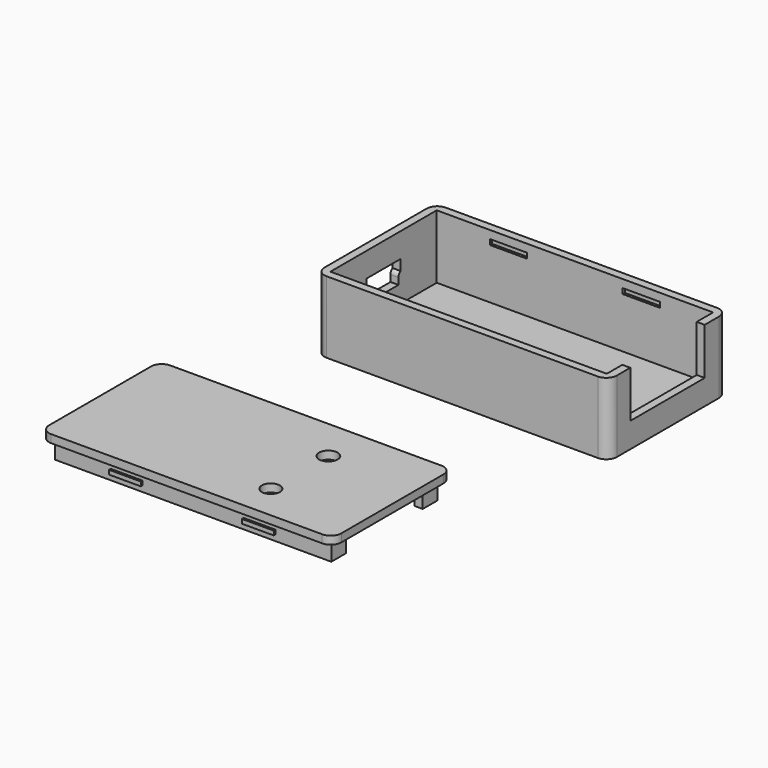
from build123d import *

# Parameters (mm, degrees)
F0_W        = 52
F0_H        = 25
F0_R        = 1.75
F1_DEPTH    = 1.5
F2_DEPTH    = 13.5
F3_W        = 17.5
F3_H        = 8.8
F4_DEPTH    = 25
F5_W        = 7
F5_H        = 2.1
F6_DEPTH    = 2
F7_T1_DEPTH = 5.8301270189
F9_W        = 7
F9_H        = 1
F10_DEPTH   = 0.5
F11_W       = 7
F11_H       = 1
F12_DEPTH   = 0.5
F0_R_2      = 1.7
F0_W_2      = 1.5
F0_H_2      = 18
F13_DEPTH   = 1.5
F14_DEPTH   = 5
F15_W       = 6
F15_H       = 0.8
F16_DEPTH   = 0.4
F17_W       = 6
F17_H       = 0.8
F18_DEPTH   = 0.5


# Not quite as in the source:
# - a fillet or chamfer that OpenCascade refuses, or shapes differently, is made with other operations: its cross-section is extruded or revolved along the edge and cut away or added


with BuildPart() as f1:
    # F0 (on Top) → F1 (new body)
    with BuildSketch(Plane.XY):
        Rectangle(F0_W, F0_H)
        with Locations((-21.9428632408, 0)):
            Circle(F0_R, mode=Mode.SUBTRACT)
        with Locations((-21.9428632408, 0)):
            Circle(F0_R)
    extrude(amount=F1_DEPTH)

    # F0 (on Top) → F2 (join)
    with BuildSketch(Plane.XY):
        with BuildLine():
            Line((25.5, 14), (-25.5, 14))
            ThreePointArc((-25.5, 14), (-26.9142135624, 13.4142135624), (-27.5, 12))
            Line((-27.5, 12), (-27.5, -12))
            ThreePointArc((-27.5, -12), (-26.9142135624, -13.4142135624), (-25.5, -14))
            Line((-25.5, -14), (25.5, -14))
            ThreePointArc((25.5, -14), (26.9142135624, -13.4142135624), (27.5, -12))
            Line((27.5, -12), (27.5, 12))
            ThreePointArc((27.5, 12), (26.9142135624, 13.4142135624), (25.5, 14))
        make_face()
        Rectangle(F0_W, F0_H, mode=Mode.SUBTRACT)
    extrude(amount=F2_DEPTH)

    # F3 (on face) → F4 (cut)
    with BuildSketch(Plane.YZ.offset(27.5)):
        with Locations((-0.1, 9.1)):
            Rectangle(F3_W, F3_H)
    extrude(amount=-F4_DEPTH, mode=Mode.SUBTRACT)

    # F5 (on face) → F6 (cut)
    with BuildSketch(Plane(origin=(-27.5, 0, 0), x_dir=(0, -1, 0), z_dir=(-1, 0, 0))):
        with Locations((0, 5.85)):
            Rectangle(F5_W, F5_H)
        Polygon((-3.5, 6.9), (3.5, 6.9), (4, 6.9), (4, 8.9), (-4, 8.9), (-4, 6.9), align=None)
    extrude(amount=-F6_DEPTH, mode=Mode.SUBTRACT)

    # F7: fillet of radius 1 on 2 edges, made by hand

    # F7_s2 → F7_t1 (cut)
    with BuildSketch(Plane.YZ.offset(-29.6650635095)):
        with BuildLine():
            ThreePointArc((3.5, 6.0339745962), (3.6339745962, 6.5339745962), (4, 6.9))
            Line((4, 6.9), (3.5, 6.9))
            Line((3.5, 6.9), (3.5, 6.0339745962))
        make_face()
        with BuildLine():
            ThreePointArc((-4, 6.9), (-3.6339745962, 6.5339745962), (-3.5, 6.0339745962))
            Line((-3.5, 6.0339745962), (-3.5, 6.9))
            Line((-3.5, 6.9), (-4, 6.9))
        make_face()
    extrude(amount=F7_T1_DEPTH, mode=Mode.SUBTRACT)

    # F9 (on face) → F10 (cut)
    with BuildSketch(Plane.XZ.offset(-12.5)):
        with Locations((-12.5, 11.5)):
            Rectangle(F9_W, F9_H)
        with Locations((12.5, 11.5)):
            Rectangle(F9_W, F9_H)
    extrude(amount=-F10_DEPTH, mode=Mode.SUBTRACT)

    # F11 (on face) → F12 (cut)
    with BuildSketch(Plane(origin=(0, -12.5, 0), x_dir=(-1, 0, 0), z_dir=(0, 1, 0))):
        with Locations((-12.5, 11.5)):
            Rectangle(F11_W, F11_H)
        with Locations((12.5, 11.5)):
            Rectangle(F11_W, F11_H)
    extrude(amount=-F12_DEPTH, mode=Mode.SUBTRACT)


with BuildPart() as f13:
    # F0 (on Top) → F13 (new body)
    with BuildSketch(Plane.XY):
        with BuildLine():
            Line((-42.439452043, -56.7449450493), (-42.439452043, -31.7449450493))
            Line((-42.439452043, -31.7449450493), (9.560547957, -31.7449450493))
            Line((9.560547957, -31.7449450493), (9.560547957, -35.2449450493))
            Line((9.560547957, -35.2449450493), (11.060547957, -35.2449450493))
            Line((11.060547957, -35.2449450493), (11.060547957, -32.2449450493))
            ThreePointArc((11.060547957, -32.2449450493), (10.4747615194, -30.8307314869), (9.060547957, -30.2449450493))
            Line((9.060547957, -30.2449450493), (-41.939452043, -30.2449450493))
            ThreePointArc((-41.939452043, -30.2449450493), (-43.3536656054, -30.8307314869), (-43.939452043, -32.2449450493))
            Line((-43.939452043, -32.2449450493), (-43.939452043, -56.2449450493))
            ThreePointArc((-43.939452043, -56.2449450493), (-43.3536656054, -57.6591586117), (-41.939452043, -58.2449450493))
            Line((-41.939452043, -58.2449450493), (9.060547957, -58.2449450493))
            ThreePointArc((9.060547957, -58.2449450493), (10.4747615194, -57.6591586117), (11.060547957, -56.2449450493))
            Line((11.060547957, -56.2449450493), (11.060547957, -53.2449450493))
            Line((11.060547957, -53.2449450493), (9.560547957, -53.2449450493))
            Line((9.560547957, -53.2449450493), (9.560547957, -56.7449450493))
            Line((9.560547957, -56.7449450493), (-42.439452043, -56.7449450493))
        make_face()
        Polygon((8.060547957, -53.2449450493), (8.060547957, -35.2449450493), (8.060547957, -33.2449450493), (-40.939452043, -33.2449450493), (-40.939452043, -55.2449450493), (8.060547957, -55.2449450493), align=None)
        with Locations((-38.3823152838, -44.2449450493)):
            Circle(F0_R, mode=Mode.SUBTRACT)
        with Locations((-5.889452043, -51.6449450493)):
            Circle(F0_R_2, mode=Mode.SUBTRACT)
        with Locations((-5.789452043, -38.2449450493)):
            Circle(F0_R, mode=Mode.SUBTRACT)
        with Locations((-38.3823152838, -44.2449450493)):
            Circle(F0_R)
        with Locations((8.810547957, -44.2449450493)):
            Rectangle(F0_W_2, F0_H_2)
        with Locations((10.310547957, -44.2449450493)):
            Rectangle(F0_W_2, F0_H_2)
    extrude(amount=-F13_DEPTH)

    # F0 (on Top) → F14 (join)
    with BuildSketch(Plane.XY):
        Polygon((9.560547957, -31.7449450493), (-42.439452043, -31.7449450493), (-42.439452043, -56.7449450493), (9.560547957, -56.7449450493), (9.560547957, -53.2449450493), (8.060547957, -53.2449450493), (8.060547957, -55.2449450493), (-40.939452043, -55.2449450493), (-40.939452043, -33.2449450493), (8.060547957, -33.2449450493), (8.060547957, -35.2449450493), (9.560547957, -35.2449450493), align=None)
    extrude(amount=-F14_DEPTH)

    # F15 (on face) → F16 (join)
    with BuildSketch(Plane.XZ.offset(56.7449450493)):
        with Locations((-28.939452043, -3.5)):
            Rectangle(F15_W, F15_H)
        with Locations((-3.939452043, -3.5)):
            Rectangle(F15_W, F15_H)
    extrude(amount=F16_DEPTH)

    # F17 (on face) → F18 (join)
    with BuildSketch(Plane(origin=(0, -31.7449450493, 0), x_dir=(-1, 0, 0), z_dir=(0, 1, 0))):
        with Locations((28.939452043, -3.2)):
            Rectangle(F17_W, F17_H)
        with Locations((3.939452043, -3.2)):
            Rectangle(F17_W, F17_H)
    extrude(amount=F18_DEPTH)


solid = Compound([f1.part, f13.part])
